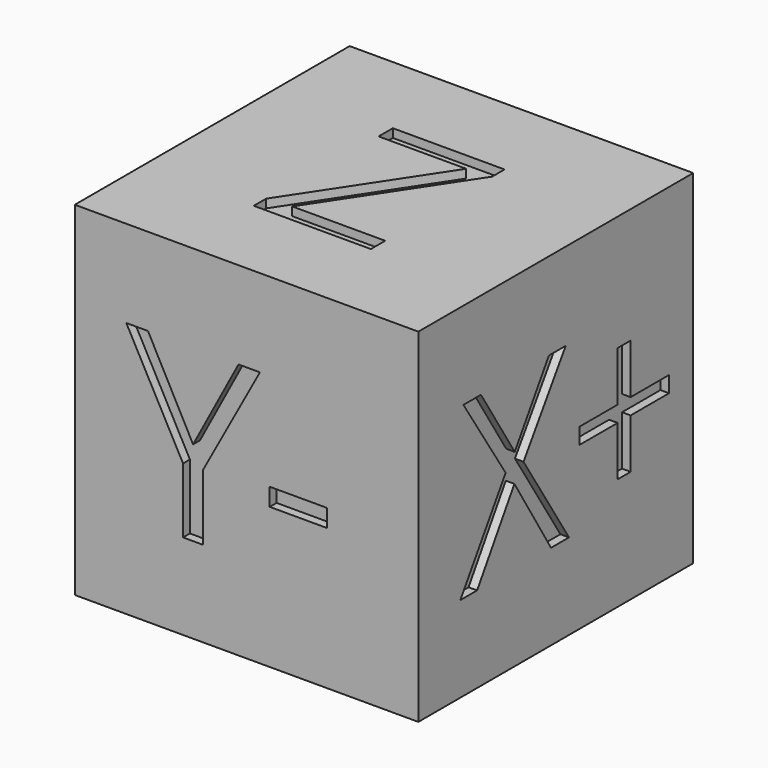
from build123d import *

# Parameters (mm, degrees)
F0_W          = 100
F0_H          = 100
F1_DEPTH      = 100
F2_TEXT_SIZE  = 69.4444444444
F3_DEPTH      = 2.5
F4_TEXT_SIZE  = 69.4444444444
F5_DEPTH      = 2.5
F6_TEXT_SIZE  = 69.4444444444
F7_DEPTH      = 2.5
F8_TEXT_SIZE  = 69.4444444444
F9_DEPTH      = 2.5
F10_TEXT_SIZE = 69.4444444444
F11_DEPTH     = 2.5


# Not quite as in the source:
# - Text() gives the source's letters only with a copy of the font that has no kerning and outlines rounded to 1/6400 em; it was checked with that copy


with BuildPart() as f1:
    # F0 (on Top) → F1 (new body)
    with BuildSketch(Plane.XY):
        with Locations((50, 50)):
            Rectangle(F0_W, F0_H)
    extrude(amount=F1_DEPTH)

    # F2 (on face) → F3 (cut)
    with BuildSketch(Plane.YZ.offset(100)):
        with Locations((15, 25)):
            Text('X+', F2_TEXT_SIZE, font='Open Sans', text_align=(TextAlign.LEFT, TextAlign.BOTTOM))
    extrude(amount=-F3_DEPTH, mode=Mode.SUBTRACT)

    # F4 (on face) → F5 (cut)
    with BuildSketch(Plane(origin=(0, 0, 0), x_dir=(0, -1, 0), z_dir=(-1, 0, 0))):
        with Locations((-85, 25)):
            Text('X-', F4_TEXT_SIZE, font='Open Sans', text_align=(TextAlign.LEFT, TextAlign.BOTTOM))
    extrude(amount=-F5_DEPTH, mode=Mode.SUBTRACT)

    # F6 (on face) → F7 (cut)
    with BuildSketch(Plane.XZ):
        with Locations((15, 25)):
            Text('Y-', F6_TEXT_SIZE, font='Open Sans', text_align=(TextAlign.LEFT, TextAlign.BOTTOM))
    extrude(amount=-F7_DEPTH, mode=Mode.SUBTRACT)

    # F8 (on face) → F9 (cut)
    with BuildSketch(Plane(origin=(0, 100, 0), x_dir=(-1, 0, 0), z_dir=(0, 1, 0))):
        with Locations((-85, 25)):
            Text('Y+', F8_TEXT_SIZE, font='Open Sans', text_align=(TextAlign.LEFT, TextAlign.BOTTOM))
    extrude(amount=-F9_DEPTH, mode=Mode.SUBTRACT)

    # F10 (on face) → F11 (cut)
    with BuildSketch(Plane.XY.offset(100)):
        with Locations((29.3185763889, 25)):
            Text('Z', F10_TEXT_SIZE, font='Open Sans', text_align=(TextAlign.LEFT, TextAlign.BOTTOM))
    extrude(amount=-F11_DEPTH, mode=Mode.SUBTRACT)


solid = f1.part
